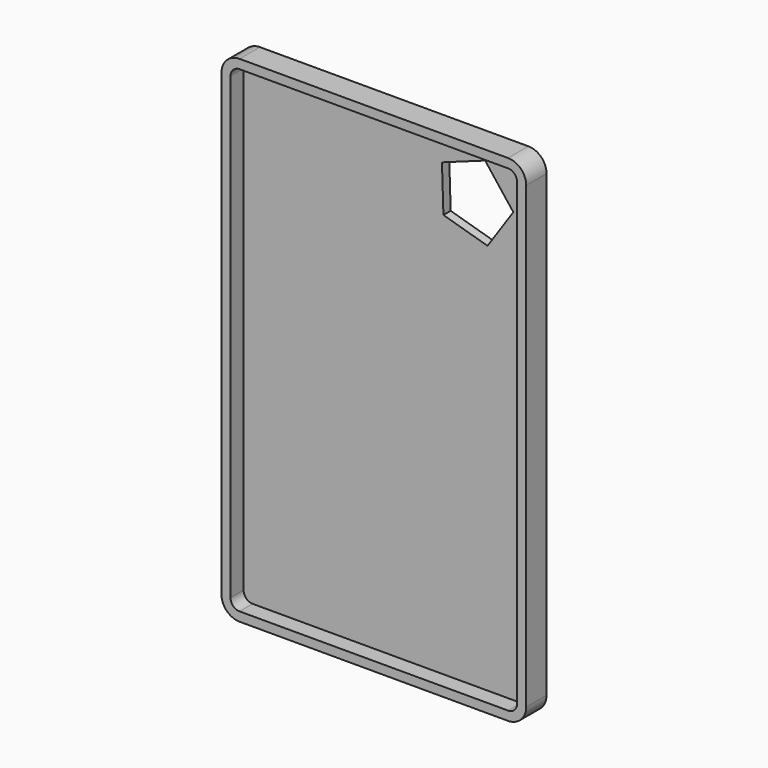
from build123d import *

# Parameters (mm, degrees)
F0_W     = 85.0665410506
F0_H     = 138.3
F1_DEPTH = 7.1
F2_R     = 5.08
F3_T     = -2.54
F5_DEPTH = 25
F8_DEPTH = 0.1


# Not quite as in the source:
# - a feature of the source that left no trace in its solid (it failed there, or was rolled back) is left out


with BuildPart() as f1:
    # F0 (on Front) → F1 (new body)
    with BuildSketch(Plane.XZ):
        Rectangle(F0_W, F0_H)
    extrude(amount=F1_DEPTH)

    # F2
    f2_edges = [f1.edges().sort_by_distance(p)[0] for p in [
        (42.533271, -3.55, -69.15),
        (-42.533271, -3.55, -69.15),
        (42.533271, -3.55, 69.15),
        (-42.533271, -3.55, 69.15),
    ]]
    fillet(f2_edges, radius=F2_R)

    # F3
    f3_openings = [f1.faces().sort_by_distance(p)[0] for p in [
        (0, -7.1, 0),
    ]]
    offset(amount=F3_T, openings=f3_openings)

    # F4 (on face) → F5 (cut)
    with BuildSketch(Plane.XZ.offset(2.54)):
        Polygon((15.775061698, 46.2421439753), (28.0853956244, 42.6747929635), (35.2822504398, 53.2802441743), (27.4198174015, 63.4021245005), (15.3637117341, 59.0523393613), align=None)
    extrude(amount=-F5_DEPTH, mode=Mode.SUBTRACT)

    # F7 (on face) → F8 (cut)
    with BuildSketch(Plane(origin=(0, 0, -69.15), x_dir=(1, 0, 0), z_dir=(0, 0, -1))):
        Polygon((2.8688537423, 1.343842895), (2.8688537423, 4.1069771897), (0.7085483604, 5.8297632436), (-1.9853083886, 5.2149080197), (-3.1841874281, 2.7254100423), (-1.9853083886, 0.235912065), (0.7085483604, -0.3789431589), align=None)
    extrude(amount=-F8_DEPTH, mode=Mode.SUBTRACT)


solid = f1.part
